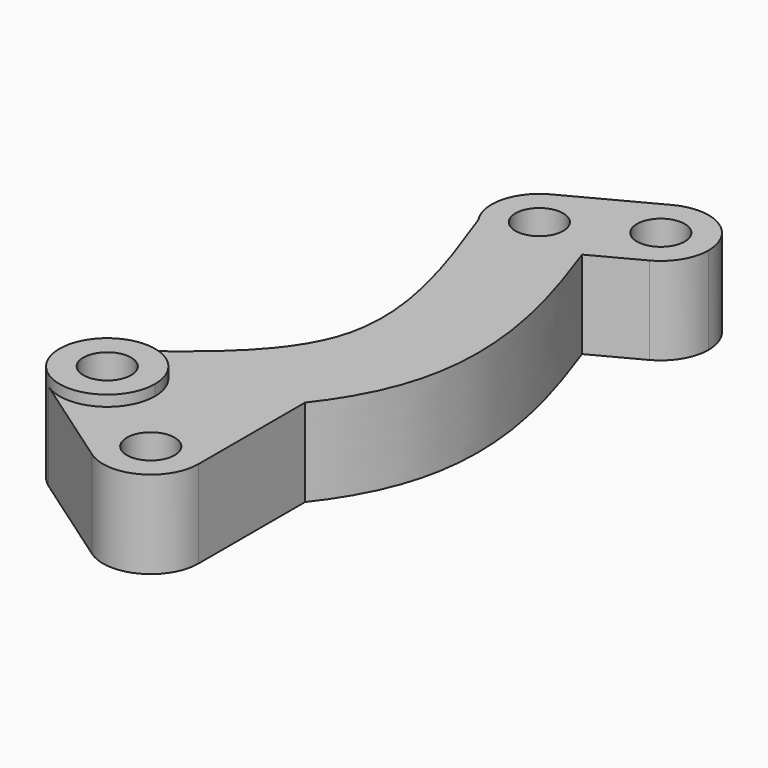
from build123d import *

# Parameters (mm, degrees)
F0_R     = 6
F1_DEPTH = 22
F2_DEPTH = 24.7


# Not quite as in the source:
# - the dataset's text gives a spline's control points without its knots; the knots are read off the source's solid
# - a feature names something its author has since deleted; it is built from what else it names


with BuildPart() as f1:
    # F0 (on Top) → F1 (new body)
    with BuildSketch(Plane.XY):
        with BuildLine():
            ThreePointArc((-44.2506901264, 54.2390673163), (-37.2170072256, 49.3508335883), (-28.7157507853, 50.3978116504))
            ThreePointArc((-28.7157507853, 50.3978116504), (-24.0543074262, 54.8133136372), (-22.3365694268, 61))
            ThreePointArc((-22.3365694268, 61), (-28.149883064, 71.2822620006), (-39.9573880683, 71.6021883496))
            ThreePointArc((-39.9573880683, 71.6021883496), (-45.9857358385, 63.8804377989), (-44.2506901264, 54.2390673163))
        make_face()
        with Locations((-34.3365694268, 61)):
            Circle(F0_R, mode=Mode.SUBTRACT)
        with BuildLine():
            ThreePointArc((-41.1910181988, -70.8496970528), (-28.7801940464, -71.6361032635), (-22.3365694268, -61))
            ThreePointArc((-22.3365694268, -61), (-39.8929448072, -50.3638967365), (-41.1910181988, -70.8496970528))
        make_face()
        with Locations((-34.3365694268, -61)):
            Circle(F0_R, mode=Mode.SUBTRACT)
        with BuildLine():
            ThreePointArc((-18.536827307, 82.9584370096), (-23.5181968435, 66.7354296949), (-7.2951893768, 61.7540606536))
            ThreePointArc((-7.2951893768, 61.7540606536), (-2.6337464761, 66.1695626111), (-0.9160086655, 72.35624866))
            ThreePointArc((-0.9160086655, 72.35624866), (-6.7293223028, 82.6385106606), (-18.536827307, 82.9584370096))
        make_face()
        with Locations((-12.9160086655, 72.35624866)):
            Circle(F0_R, mode=Mode.SUBTRACT)
        with BuildLine():
            Line((-22.3365694268, 51.1162809556), (-22.3365694268, -27.5282078784))
            add(Edge.make_bspline(
                [(-19.1679852382, 55.4596212318), (-19.1490913177, 55.4067702681), (-18.2627780559, 52.9264771043), (-16.5142433132, 47.9330355336), (-14.0597955985, 40.2848666723), (-11.8817933237, 32.380636116), (-10.1403594344, 24.1713941631), (-9.0428174028, 15.5795000988), (-8.9070069048, 8.0286707772), (-9.4009784523, 2.5365834769), (-9.8823537024, -0.64961691), (-10.3506440426, -3.0593767725), (-10.9326328555, -5.4817632435), (-11.6386397696, -7.9166705081), (-12.4443293031, -10.2769526895), (-13.6414482379, -13.3297795407), (-15.3453349713, -16.9551929086), (-17.6521060756, -20.9929507786), (-20.005676914, -24.5007883382), (-21.6047261121, -26.6086284401), (-22.3365694268, -27.5282078784)],
                knots=[0.0611387127, 0.0611387127, 0.0611387127, 0.0611387127, 0.0625, 0.125, 0.1875, 0.25, 0.3125, 0.375, 0.4375, 0.46875, 0.484375, 0.5, 0.515625, 0.53125, 0.546875, 0.5625, 0.59375, 0.625, 0.65625, 0.6818147445, 0.6818147445, 0.6818147445, 0.6818147445], degree=3))
            Line((-19.1679852382, 55.4596212318), (-21.0545147962, 54.4594654001))
            ThreePointArc((-21.0545147962, 54.4594654001), (-22.0050663394, 52.9065704787), (-22.3365694268, 51.1162809556))
        make_face()
        with BuildLine():
            ThreePointArc((-41.1910181988, -70.8496970528), (-39.8929448072, -50.3638967365), (-22.3365694268, -61))
            Line((-22.3365694268, -61), (-22.3365694268, -27.5282078784))
            Line((-22.3365694268, -27.5282078784), (-22.3365694268, 51.1162809556))
            ThreePointArc((-22.3365694268, 51.1162809556), (-22.0050663394, 52.9065704787), (-21.0545147962, 54.4594654001))
            Line((-21.0545147962, 54.4594654001), (-28.7157507853, 50.3978116504))
            ThreePointArc((-28.7157507853, 50.3978116504), (-37.2170072256, 49.3508335883), (-44.2506901264, 54.2390673163))
            add(Edge.make_bspline(
                [(-44.2506901264, 54.2390673163), (-37.1132332482, 34.6511342855), (-23.4734527351, -2.7816813244), (-51.824990918, -23.6902906337), (-65.3406685812, -33.657792996)],
                knots=[0, 0, 0, 0, 0.523282385, 1, 1, 1, 1], degree=3))
            ThreePointArc((-65.3406685812, -33.657792996), (-53.1694343986, -33.3492849771), (-46.993012785, -43.8414694388))
            ThreePointArc((-46.993012785, -43.8414694388), (-53.4366374046, -54.4775727023), (-65.847461557, -53.6911664916))
            Line((-65.847461557, -53.6911664916), (-41.1910181988, -70.8496970528))
        make_face()
        with BuildLine():
            Line((-21.0545147962, 54.4594654001), (-19.1679852382, 55.4596212318))
            Line((-19.1679852382, 55.4596212318), (-7.2951893768, 61.7540606536))
            ThreePointArc((-7.2951893768, 61.7540606536), (-23.5181968435, 66.7354296949), (-18.536827307, 82.9584370096))
            Line((-18.536827307, 82.9584370096), (-39.9573880683, 71.6021883496))
            ThreePointArc((-39.9573880683, 71.6021883496), (-28.149883064, 71.2822620006), (-22.3365694268, 61))
            ThreePointArc((-22.3365694268, 61), (-24.0543074262, 54.8133136372), (-28.7157507853, 50.3978116504))
            Line((-28.7157507853, 50.3978116504), (-21.0545147962, 54.4594654001))
        make_face()
    extrude(amount=F1_DEPTH)

    # F0 (on Top) → F2 (join)
    with BuildSketch(Plane.XY):
        with BuildLine():
            ThreePointArc((-70.6743202458, -41.0942788729), (-70.1985453114, -48.1351905289), (-65.847461557, -53.6911664916))
            ThreePointArc((-65.847461557, -53.6911664916), (-53.4366374046, -54.4775727023), (-46.993012785, -43.8414694388))
            ThreePointArc((-46.993012785, -43.8414694388), (-53.1694343986, -33.3492849771), (-65.3406685812, -33.657792996))
            ThreePointArc((-65.3406685812, -33.657792996), (-68.7442285851, -36.8476299769), (-70.6743202458, -41.0942788729))
        make_face()
        with Locations((-58.993012785, -43.8414694388)):
            Circle(F0_R, mode=Mode.SUBTRACT)
    extrude(amount=F2_DEPTH)


solid = f1.part
